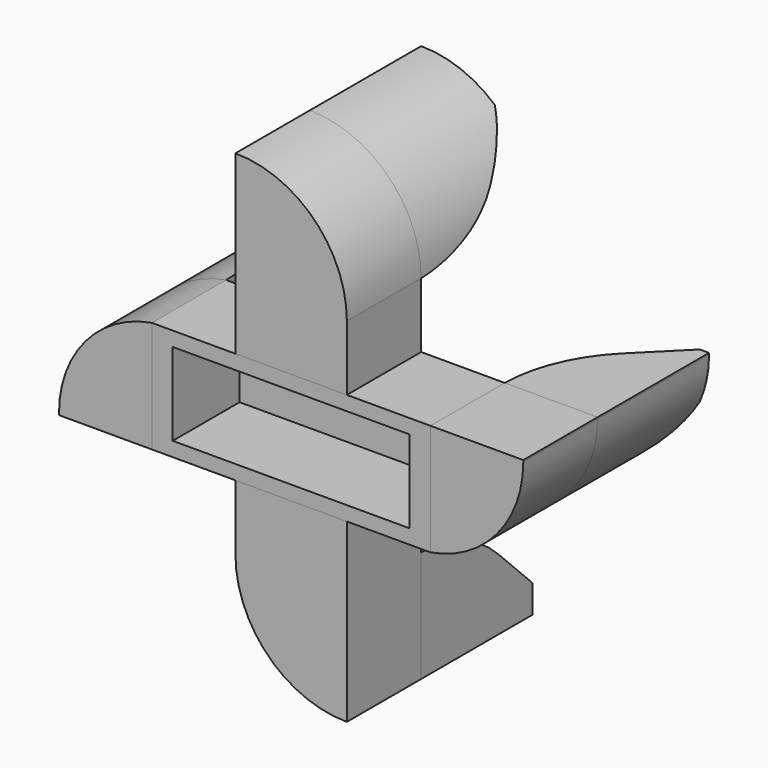
from build123d import *

# Parameters (mm, degrees)
F0_W            = 25.5
F0_H            = 8.9
F1_DEPTH        = 8.9
F2_W            = 30
F2_H            = 12
F2_W_2          = 25.5
F2_H_2          = 8.9
F3_DEPTH        = 10
F4_DEPTH        = 9
F5_DEPTH        = 10
F6_DEPTH        = 10
F8_DEPTH        = 19
F10_DEPTH       = 19
F11_T1_DEPTH    = 69.160797831
F11_2_T1_DEPTH  = 69.160797831
F11_3_T1_DEPTH  = 70
F11_4_T1_DEPTH  = 70
F13_DEPTH       = 15
F14_SIZE        = 9
F15_T1_DEPTH    = 43.0551475556
F15_S1_T1_DEPTH = 43.0551475556
F15_S2_T1_DEPTH = 43.0551475556
F15_S3_T1_DEPTH = 43.0551475556


# Not quite as in the source:
# - a fillet or chamfer that OpenCascade refuses, or shapes differently, is made with other operations: its cross-section is extruded or revolved along the edge and cut away or added


with BuildPart() as f1:
    # F0 (on Top) → F1 (new body)
    with BuildSketch(Plane.XY):
        with Locations((12.75, 4.45)):
            Rectangle(F0_W, F0_H)
    extrude(amount=F1_DEPTH)


with BuildPart() as f3:
    # F2 (on face) → F3 (new body)
    with BuildSketch(Plane.XZ):
        with Locations((12.75, 4.45)):
            Rectangle(F2_W, F2_H)
        with Locations((12.75, 4.45)):
            Rectangle(F2_W_2, F2_H_2, mode=Mode.SUBTRACT)
        with Locations((12.75, 4.45)):
            Rectangle(F2_W_2, F2_H_2)
    extrude(amount=-F3_DEPTH)


with BuildPart() as f4_tool:
    # F4 (cut): a face of the model
    f4_faces = [f1.part.faces().sort_by_distance(p)[0] for p in [
        (12.75, 0, 4.45),
    ]]
    extrude(f4_faces, amount=-F4_DEPTH)


with BuildPart() as f1_1:
    add(f1.part)

    # F4: cut by f4_tool
    add(f4_tool.part, mode=Mode.SUBTRACT)


with BuildPart() as f3_1:
    add(f3.part)

    # F4: cut by f4_tool
    add(f4_tool.part, mode=Mode.SUBTRACT)


with BuildPart() as f5:
    # F5 (new): a face of the model
    f5_faces = [f3_1.part.faces().sort_by_distance(p)[0] for p in [
        (-2.25, 5, 4.45),
    ]]
    extrude(f5_faces, amount=F5_DEPTH)

    # F11: fillet of radius 12 on 1 edges, made by hand

    # F11_s2 → F11_t1 (cut)
    with BuildSketch(Plane.XZ.offset(-39.5803989155)):
        with BuildLine():
            ThreePointArc((-2.25, 10.45), (-9.4151513899, 6.3638071262), (-12.25, -1.3821595662))
            Line((-12.25, -1.3821595662), (-12.25, 10.45))
            Line((-12.25, 10.45), (-2.25, 10.45))
        make_face()
    extrude(amount=F11_T1_DEPTH, mode=Mode.SUBTRACT)


with BuildPart() as f6:
    # F6 (new): a face of the model
    f6_faces = [f3_1.part.faces().sort_by_distance(p)[0] for p in [
        (27.75, 5, 4.45),
    ]]
    extrude(f6_faces, amount=F6_DEPTH)

    # F11#2: fillet of radius 12 on 1 edges, made by hand

    # F11_2_s2 → F11_2_t1 (cut)
    with BuildSketch(Plane.XZ.offset(-39.5803989155)):
        with BuildLine():
            ThreePointArc((27.75, -1.55), (34.9151513899, 2.5361928738), (37.75, 10.2821595662))
            Line((37.75, 10.2821595662), (37.75, -1.55))
            Line((37.75, -1.55), (27.75, -1.55))
        make_face()
    extrude(amount=F11_2_T1_DEPTH, mode=Mode.SUBTRACT)


with BuildPart() as f8:
    # F7 (on face) → F8 (new body)
    with BuildSketch(Plane.XY.offset(10.45)):
        Polygon((6.75, 0), (12.75, 0), (18.75, 0), (18.75, 10), (12.75, 10), (6.75, 10), align=None)
    extrude(amount=F8_DEPTH)

    # F11#3: fillet of radius 12 on 1 edges, made by hand

    # F11_3_s2 → F11_3_t1 (cut)
    with BuildSketch(Plane.XZ.offset(-40)):
        with BuildLine():
            ThreePointArc((18.75, 17.45), (15.2352813742, 25.9352813742), (6.75, 29.45))
            Line((6.75, 29.45), (18.75, 29.45))
            Line((18.75, 29.45), (18.75, 17.45))
        make_face()
    extrude(amount=F11_3_T1_DEPTH, mode=Mode.SUBTRACT)


with BuildPart() as f10:
    # F9 (on face) → F10 (new body)
    with BuildSketch(Plane(origin=(0, 0, -1.55), x_dir=(1, 0, 0), z_dir=(0, 0, -1))):
        Polygon((6.75, -10), (12.75, -10), (18.75, -10), (18.75, 0), (12.75, 0), (6.75, 0), align=None)
    extrude(amount=F10_DEPTH)

    # F11#4: fillet of radius 12 on 1 edges, made by hand

    # F11_4_s2 → F11_4_t1 (cut)
    with BuildSketch(Plane.XZ.offset(-40)):
        with BuildLine():
            ThreePointArc((18.75, -20.55), (10.2647186258, -17.0352813742), (6.75, -8.55))
            Line((6.75, -8.55), (6.75, -20.55))
            Line((6.75, -20.55), (18.75, -20.55))
        make_face()
    extrude(amount=F11_4_T1_DEPTH, mode=Mode.SUBTRACT)


with BuildPart() as f13:
    # F12 (on face) + F6_face (on face) + F5_face (on face) → F13 (new body)
    with BuildSketch(Plane(origin=(0, 10, 0), x_dir=(-1, 0, 0), z_dir=(0, 1, 0))):
        with BuildLine():
            Line((-6.75, -8.55), (-18.75, -8.55))
            Line((-18.75, -8.55), (-18.75, -20.55))
            ThreePointArc((-18.75, -20.55), (-10.2647186258, -17.0352813742), (-6.75, -8.55))
        make_face()
        with BuildLine():
            ThreePointArc((-6.75, 29.45), (-15.2352813742, 25.9352813742), (-18.75, 17.45))
            Line((-18.75, 17.45), (-6.75, 17.45))
            Line((-6.75, 17.45), (-6.75, 29.45))
        make_face()
    with BuildSketch(Plane(origin=(31.9545650096, 10, 5.515900775), x_dir=(-1, 0, 0), z_dir=(0, 1, 0))):
        with BuildLine():
            Line((4.2045650096, -7.065900775), (4.2045650096, 4.934099225))
            Line((4.2045650096, 4.934099225), (-5.7954349904, 4.934099225))
            Line((-5.7954349904, 4.934099225), (-5.7954349904, 4.7662587912))
            ThreePointArc((-5.7954349904, 4.7662587912), (-2.9605863803, -2.9797079012), (4.2045650096, -7.065900775))
        make_face()
    with BuildSketch(Plane(origin=(-6.4545650096, 10, 3.384099225), x_dir=(-1, 0, 0), z_dir=(0, 1, 0))):
        with BuildLine():
            Line((-4.2045650096, 7.065900775), (-4.2045650096, -4.934099225))
            Line((-4.2045650096, -4.934099225), (5.7954349904, -4.934099225))
            Line((5.7954349904, -4.934099225), (5.7954349904, -4.7662587912))
            ThreePointArc((5.7954349904, -4.7662587912), (2.9605863803, 2.9797079012), (-4.2045650096, 7.065900775))
        make_face()
    extrude(amount=F13_DEPTH)

    # F14
    f14_edges = [f13.edges().sort_by_distance(p)[0] for p in [
        (-2.25, 25, 4.45),
        (12.75, 25, 17.45),
        (27.75, 25, 4.45),
        (12.75, 25, -8.55),
    ]]
    chamfer(f14_edges, length=F14_SIZE)

    # F15: fillet of radius 15 on 1 edges, made by hand

    # F15_s2 → F15_t1 (cut)
    with BuildSketch(Plane.XY.offset(-17.0775737778)):
        with BuildLine():
            ThreePointArc((-2.25, 10), (-3.4317147602, 15.6245635654), (-6.6418610855, 20.3918610855))
            Line((-6.6418610855, 20.3918610855), (-2.25, 16))
            Line((-2.25, 16), (-2.25, 10))
        make_face()
    extrude(amount=F15_T1_DEPTH, mode=Mode.SUBTRACT)

    # F15#s1: fillet of radius 15 on 1 edges, made by hand

    # F15_s1_s2 → F15_s1_t1 (cut)
    with BuildSketch(Plane.YZ.offset(-8.7775737778)):
        with BuildLine():
            ThreePointArc((10, 17.45), (15.6245635654, 18.6317147602), (20.3918610855, 21.8418610855))
            Line((20.3918610855, 21.8418610855), (16, 17.45))
            Line((16, 17.45), (10, 17.45))
        make_face()
    extrude(amount=F15_S1_T1_DEPTH, mode=Mode.SUBTRACT)

    # F15#s2: fillet of radius 15 on 1 edges, made by hand

    # F15_s2_s2 → F15_s2_t1 (cut)
    with BuildSketch(Plane.XY.offset(-17.0775737778)):
        with BuildLine():
            ThreePointArc((27.75, 10), (28.9317147602, 15.6245635654), (32.1418610855, 20.3918610855))
            Line((32.1418610855, 20.3918610855), (27.75, 16))
            Line((27.75, 16), (27.75, 10))
        make_face()
    extrude(amount=F15_S2_T1_DEPTH, mode=Mode.SUBTRACT)

    # F15#s3: fillet of radius 15 on 1 edges, made by hand

    # F15_s3_s2 → F15_s3_t1 (cut)
    with BuildSketch(Plane.YZ.offset(-8.7775737778)):
        with BuildLine():
            ThreePointArc((10, -8.55), (15.6245635654, -9.7317147602), (20.3918610855, -12.9418610855))
            Line((20.3918610855, -12.9418610855), (16, -8.55))
            Line((16, -8.55), (10, -8.55))
        make_face()
    extrude(amount=F15_S3_T1_DEPTH, mode=Mode.SUBTRACT)


solid = Compound([f3_1.part, f5.part, f6.part, f8.part, f10.part, f13.part])
